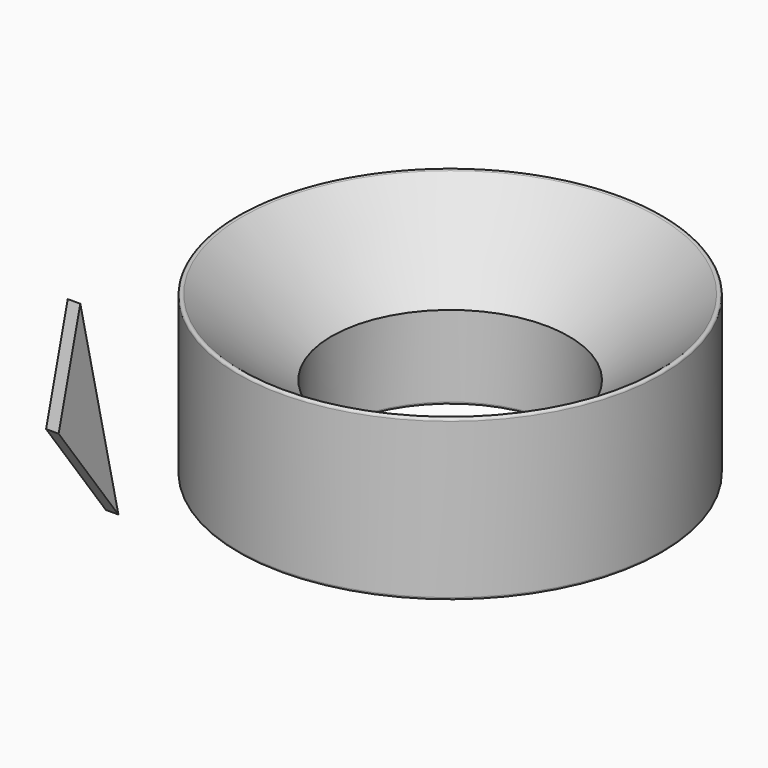
from build123d import *

# Parameters (mm, degrees)
F0_W     = 165.3737425804
F0_H     = 124.4190223515
F1_DEPTH = 25.4
F3_W     = 115.6221553683
F3_H     = 126.1607408524
F3_W_2   = 170.5438941717
F3_H_2   = 219.3448096514
F4_T     = -2.54
F4_2_T   = -2.54
F6_DEPTH = 25.4
F7_W     = 189.3875896931
F7_H     = 169.002037769
F9_R     = 5.08
F10_T    = -2.54


# Not quite as in the source:
# - a shell that OpenCascade refuses in one call is made with other operations: the cavity is built on its own and cut out


with BuildPart() as f1:
    # F0 (on Front) → F1 (new body)
    with BuildSketch(Plane.XZ):
        with Locations((-11.4489495754, -2.2449400276)):
            Rectangle(F0_W, F0_H)
    extrude(amount=F1_DEPTH)

    # F3 (on Right) → F11, piece 2 (revolve)
    with BuildSketch(Plane.YZ):
        with Locations((100.368924439, 45.5251559615)):
            Rectangle(F3_W_2, F3_H_2)
    revolve(axis=Axis((71.2379217148, -25.4, -2.2449400276), (0, 0, -1)))

    # F4#2
    f4_2_openings = [f1.faces().sort_by_distance(p)[0] for p in [
        (140.460931, -230.471734, 155.197561),
    ]]
    offset(amount=F4_2_T, openings=f4_2_openings, kind=Kind.INTERSECTION)


with BuildPart() as f11:
    # F3 (on Right) → F11 (revolve)
    with BuildSketch(Plane.YZ):
        with Locations((128.4491606057, 218.544781208)):
            Rectangle(F3_W, F3_H)
    revolve(axis=Axis((71.2379217148, -25.4, -2.2449400276), (0, 0, -1)))

    # F4
    f4_openings = [f11.faces().sort_by_distance(p)[0] for p in [
        (140.460931, -231.073583, 281.625152),
    ]]
    offset(amount=F4_T, openings=f4_openings)


with BuildPart() as f6:
    # F2 (on Right) → F6 (new body)
    with BuildSketch(Plane.YZ):
        Polygon((-162.2416079044, 209.2569768429), (-217.0603871346, 0), (-65.8233910799, -205.5934518576), align=None)
    extrude(amount=F6_DEPTH)


with BuildPart() as f8:
    # F7 (on Front) → F8 (revolve)
    with BuildSketch(Plane.XZ):
        with Locations((309.2453479767, 123.9695076462)):
            Rectangle(F7_W, F7_H)
        Polygon((214.5515531301, 208.4705265307), (403.9391428232, 208.4705265307), (214.5515531301, 369.3135349012), align=None)
    revolve(axis=Axis((644.0016031265, 0, 168.0627539754), (0, 0, -1)))

    # F9
    f9_edges = [f8.edges().sort_by_distance(p)[0] for p in [
        (1073.451653, 0, 369.313535),
        (1073.451653, 0, 39.468489),
        (884.064063, 0, 39.468489),
    ]]
    fillet(f9_edges, radius=F9_R)

    # F10: a shell. OpenCascade refuses it in one call, so the cavity is built on its own and cut out:
    # the body offset inwards by the wall thickness, plus a prism from it out through each open face.
    f10_core = offset(f8.part, amount=F10_T, mode=Mode.PRIVATE)
    f10_exits = [f10_core.faces().sort_by_distance(p)[0] for p in [
        (1056.368656, 0, 42.008489),
    ]]
    add(f10_core, mode=Mode.SUBTRACT)
    extrude(f10_exits, amount=-F10_T, mode=Mode.SUBTRACT)


solid = Compound([f6.part, f8.part])
